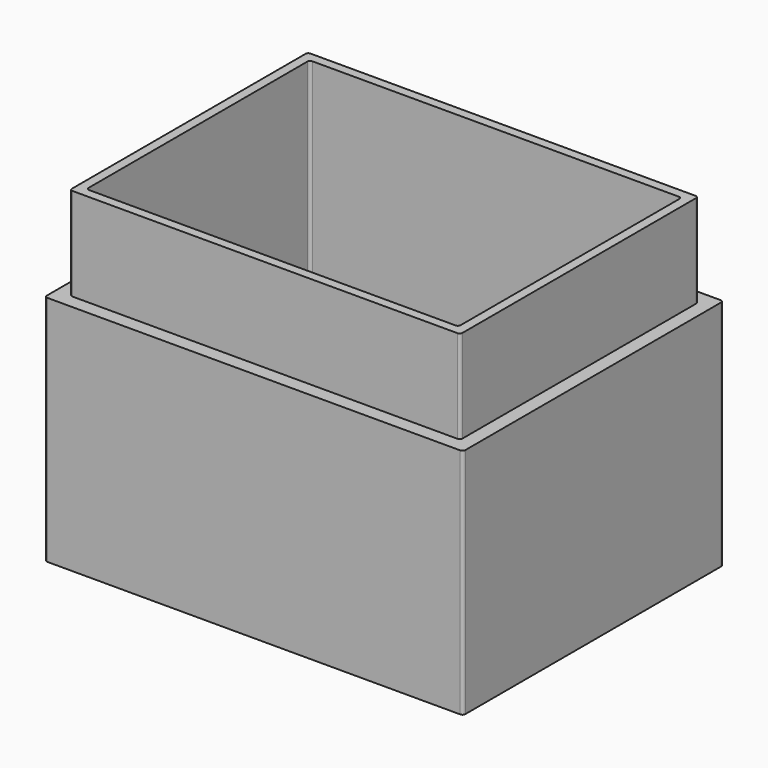
from build123d import *

# Parameters (mm, degrees)
F0_W     = 45
F0_H     = 35
F1_DEPTH = 35
F2_W     = 40
F2_H     = 30
F3_DEPTH = 30
F4_W     = 45
F4_H     = 35
F4_W_2   = 42
F4_H_2   = 32
F5_DEPTH = 10
F6_R     = 0.3


with BuildPart() as f1:
    # F0 (on Top) → F1 (new body)
    with BuildSketch(Plane.XY):
        Rectangle(F0_W, F0_H)
    extrude(amount=F1_DEPTH)

    # F2 (on face) → F3 (cut)
    with BuildSketch(Plane.XY.offset(35)):
        Rectangle(F2_W, F2_H)
    extrude(amount=-F3_DEPTH, mode=Mode.SUBTRACT)

    # F4 (on face) → F5 (cut)
    with BuildSketch(Plane.XY.offset(35)):
        Rectangle(F4_W, F4_H)
        Rectangle(F4_W_2, F4_H_2, mode=Mode.SUBTRACT)
    extrude(amount=-F5_DEPTH, mode=Mode.SUBTRACT)

    # F6
    f6_edges = [f1.edges().sort_by_distance(p)[0] for p in [
        (-22.5, 17.5, 12.5),
        (22.5, 17.5, 12.5),
        (22.5, -17.5, 12.5),
        (-22.5, -17.5, 12.5),
        (-21, -16, 30),
        (21, -16, 30),
        (21, 16, 30),
        (-21, 16, 30),
        (-20, 15, 20),
        (20, 15, 20),
        (20, -15, 20),
        (-20, -15, 20),
    ]]
    fillet(f6_edges, radius=F6_R)


solid = f1.part
